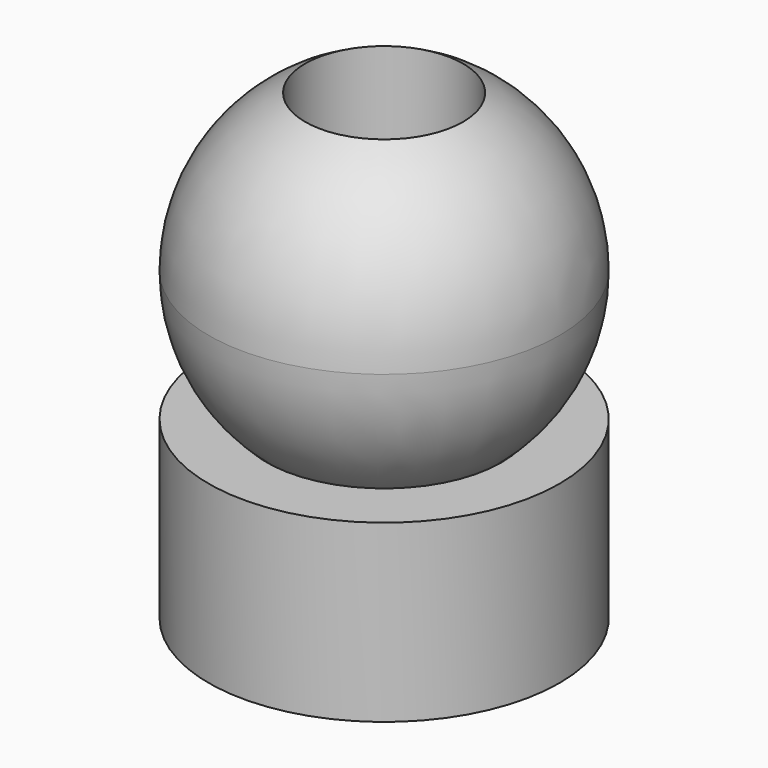
from build123d import *

# Parameters (mm, degrees)
F0_R     = 5
F0_R_2   = 1.75
F1_DEPTH = 5
F2_SIZE  = 1.6
F4_R     = 5
F4_R_2   = 2.25
F5_DEPTH = 5
F6_R     = 4.99999
F7_DEPTH = 10


# Not quite as in the source:
# - a fillet or chamfer is up to 0.001 mm smaller than in the source, because OpenCascade refuses the exact size


with BuildPart() as f1:
    # F0 (on Top) → F1 (new body)
    with BuildSketch(Plane.XY):
        Circle(F0_R)
        Circle(F0_R_2, mode=Mode.SUBTRACT)
    extrude(amount=F1_DEPTH)

    # F2
    f2_edges = [f1.edges().sort_by_distance(p)[0] for p in [
        (-1.75, 0, 5),
    ]]
    chamfer(f2_edges, length=F2_SIZE)


with BuildPart() as f5:
    # F4 (on offset) → F5 (new body, symmetric)
    with BuildSketch(Plane.XY.offset(8.721)):
        Circle(F4_R)
        Circle(F4_R_2, mode=Mode.SUBTRACT)
        Circle(F4_R_2)
    extrude(amount=F5_DEPTH, both=True)

    # F6 (radius 5 in the source; OpenCascade refuses exactly that, so slightly less here)
    f6_edges = [f5.edges().sort_by_distance(p)[0] for p in [
        (-5, 0, 3.721),
        (5, 0, 8.721),
        (-5, 0, 13.721),
    ]]
    fillet(f6_edges, radius=F6_R)

    # F4 (on offset) → F7 (cut)
    with BuildSketch(Plane.XY.offset(8.721)):
        Circle(F4_R_2)
    extrude(amount=F7_DEPTH, mode=Mode.SUBTRACT)


solid = Compound([f1.part, f5.part])
